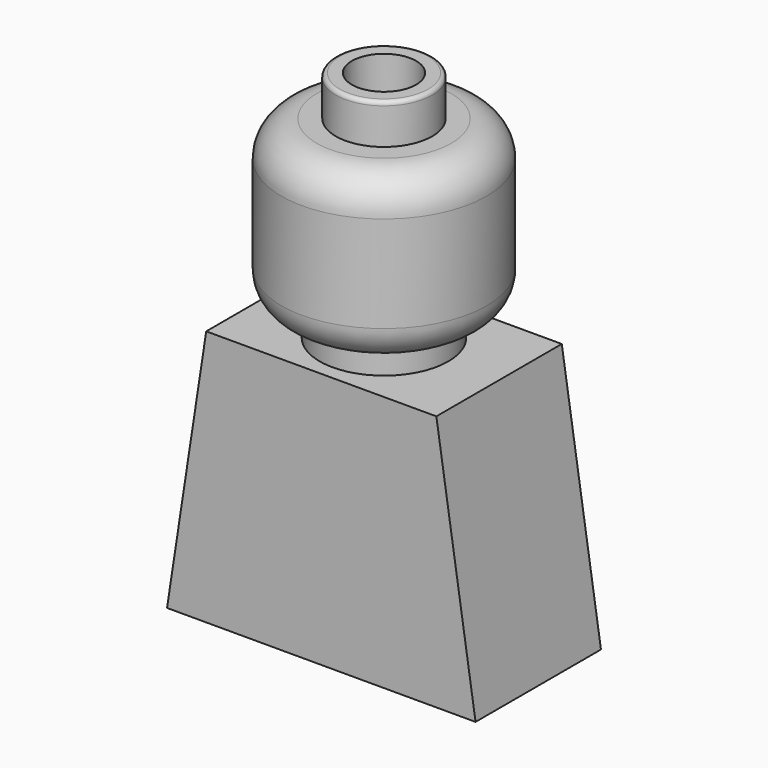
from build123d import *

# Parameters (mm, degrees)
F3_DEPTH  = 25
F4_R      = 2.4
F5_DEPTH  = 5.8
F7_DEPTH  = 3.9
F8_T      = -1.35
F10_DEPTH = 11.4


with BuildPart() as f1:
    # F0 (on Front) → F1 (revolve)
    with BuildSketch(Plane.XZ):
        with BuildLine():
            Line((0, 9.6), (0, 8.6))
            Line((0, 8.6), (2.5, 8.6))
            Line((2.5, 8.6), (2.5, 0))
            Line((2.5, 0), (3.2, 0))
            Line((3.2, 0), (3.2, 1.3))
            Line((3.2, 1.3), (3.35, 1.3))
            ThreePointArc((3.35, 1.3), (4.5874368671, 1.8125631329), (5.1, 3.05))
            Line((5.1, 3.05), (5.1, 7.85))
            ThreePointArc((5.1, 7.85), (4.5874368671, 9.0874368671), (3.35, 9.6))
            Line((3.35, 9.6), (2.4, 9.6))
            Line((2.4, 9.6), (2.4, 11.4))
            ThreePointArc((2.4, 11.4), (2.3414213562, 11.5414213562), (2.2, 11.6))
            Line((2.2, 11.6), (1.6, 11.6))
            Line((1.6, 11.6), (1.6, 9.6))
            Line((1.6, 9.6), (0, 9.6))
        make_face()
    revolve(axis=Axis((0, 0, 5.8), (0, 0, 1)))

    # F2 (on face) → F3 (cut)
    with BuildSketch(Plane.XY.offset(9.6)):
        with BuildLine():
            Line((-1.5491933385, 0.4), (-0.2309401077, 0.4))
            Line((-0.2309401077, 0.4), (0.4281865077, 1.5416407865))
            ThreePointArc((0.4281865077, 1.5416407865), (-0.8, 1.3856406461), (-1.5491933385, 0.4))
        make_face()
        with BuildLine():
            Line((1.1210068308, 1.1416407865), (0.4618802154, 0))
            Line((0.4618802154, 0), (1.1210068308, -1.1416407865))
            ThreePointArc((1.1210068308, -1.1416407865), (1.4754001032, -0.6190270878), (1.6, 0))
            ThreePointArc((1.6, 0), (1.4754001032, 0.6190270878), (1.1210068308, 1.1416407865))
        make_face()
        with BuildLine():
            Line((0.4281865077, -1.5416407865), (-0.2309401077, -0.4))
            Line((-0.2309401077, -0.4), (-1.5491933385, -0.4))
            ThreePointArc((-1.5491933385, -0.4), (-0.8, -1.3856406461), (0.4281865077, -1.5416407865))
        make_face()
    extrude(amount=-F3_DEPTH, mode=Mode.SUBTRACT)


with BuildPart() as f5:
    # F4 (on face) → F5 (new body)
    with BuildSketch(Plane(origin=(0, 0, 0), x_dir=(1, 0, 0), z_dir=(0, 0, -1))):
        Circle(F4_R)
    extrude(amount=-F5_DEPTH)

    # F6 (on Front) → F7 (join, symmetric)
    with BuildSketch(Plane.XZ):
        Polygon((5.725, 0), (0, 0), (-5.725, 0), (-7.675, -12.75), (7.675, -12.75), align=None)
    extrude(amount=F7_DEPTH, both=True)

    # F8
    f8_openings = [f5.faces().sort_by_distance(p)[0] for p in [
        (0, 0, -12.75),
    ]]
    offset(amount=F8_T, openings=f8_openings, kind=Kind.INTERSECTION)

    # F9 (on face) → F10 (join, through all)
    with BuildSketch(Plane(origin=(0, 0, -1.35), x_dir=(1, 0, 0), z_dir=(0, 0, -1))):
        Polygon((-1.625, 1.95), (-1.625, 2.55), (-2.225, 2.55), align=None)
        Polygon((2.225, 2.55), (1.625, 2.55), (1.625, 1.95), align=None)
        Polygon((-2.225, -2.55), (-1.625, -2.55), (-1.625, -1.95), align=None)
        Polygon((1.625, -1.95), (1.625, -2.55), (2.225, -2.55), align=None)
    extrude(amount=F10_DEPTH)


solid = Compound([f1.part, f5.part])
